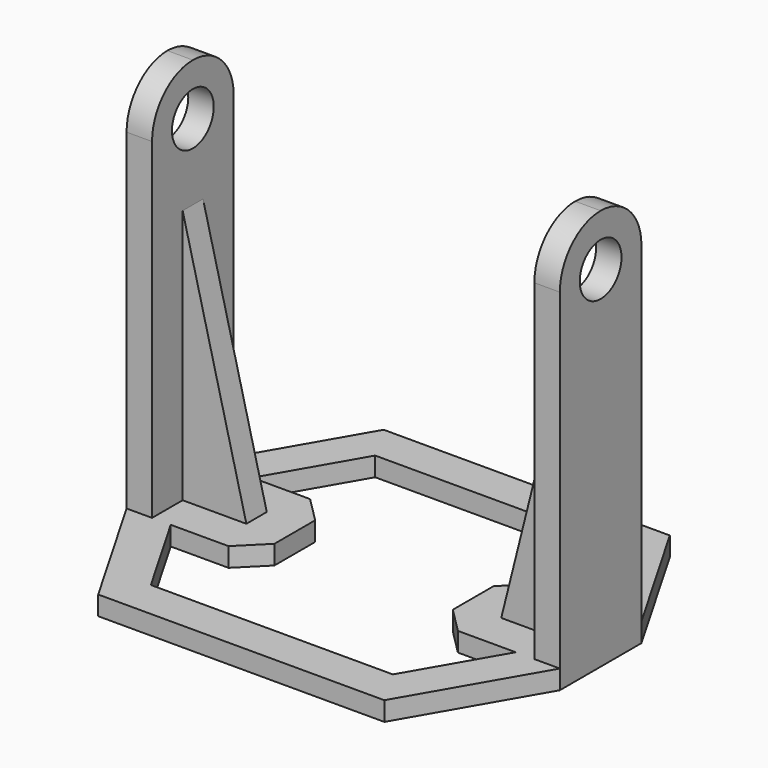
from build123d import *

# Parameters (mm, degrees)
F1_DEPTH = 4
F2_R     = 2.05
F3_DEPTH = 34.001
F5_DEPTH = 1
F7_DEPTH = 1.5
F9_DEPTH = 1.501
F10_SIZE = 2
F11_R    = 3.99999


# Not quite as in the source:
# - a fillet or chamfer is up to 0.001 mm smaller than in the source, because OpenCascade refuses the exact size


with BuildPart() as f1:
    # F0 (on Front) → F1 (new body, symmetric)
    with BuildSketch(Plane.XZ):
        Polygon((15, 0), (0, 0), (-15, 0), (-15, 30), (-17, 30), (-17, -1.5), (0, -1.5), (17, -1.5), (17, 30), (15, 30), align=None)
    extrude(amount=F1_DEPTH, both=True)

    # F2 (on face) → F3 (cut, through all)
    with BuildSketch(Plane.YZ.offset(17)):
        with Locations((0, 25.95)):
            Circle(F2_R)
    extrude(amount=-F3_DEPTH, mode=Mode.SUBTRACT)

    # F4 (on Front) → F5 (join, symmetric)
    with BuildSketch(Plane.XZ):
        Polygon((-10, 0), (-15, 20), (-15, 0), align=None)
        Polygon((15, 20), (10, 0), (15, 0), align=None)
    extrude(amount=F5_DEPTH, both=True)

    # F6 (on face) → F7 (join, through all)
    with BuildSketch(Plane.XY):
        Polygon((15, -4), (-15, -4), (-17, -4), (-11.2264973081, -14), (0, -14), (11.2264973081, -14), (17, -4), align=None)
        Polygon((-11.2264973081, 14), (-17, 4), (-15, 4), (15, 4), (17, 4), (11.2264973081, 14), (0, 14), align=None)
    extrude(amount=-F7_DEPTH)

    # F8 (on face) → F9 (cut, through all)
    with BuildSketch(Plane.XY):
        Polygon((-7, -4), (-13.5358983849, -4), (-9.4944465005, -11), (9.4944465005, -11), (13.5358983849, -4), (7, -4), (7, 4), (13.5358983849, 4), (9.4944465005, 11), (-9.4944465005, 11), (-13.5358983849, 4), (-7, 4), align=None)
    extrude(amount=-F9_DEPTH, mode=Mode.SUBTRACT)

    # F10
    f10_edges = [f1.edges().sort_by_distance(p)[0] for p in [
        (-7, -4, -0.75),
        (-7, 4, -0.75),
        (7, -4, -0.75),
        (7, 4, -0.75),
    ]]
    chamfer(f10_edges, length=F10_SIZE)

    # F11 (radius 4 in the source; OpenCascade refuses exactly that, so slightly less here)
    f11_edges = [f1.edges().sort_by_distance(p)[0] for p in [
        (-16, -4, 30),
        (16, -4, 30),
        (16, 4, 30),
        (-16, 4, 30),
    ]]
    fillet(f11_edges, radius=F11_R)


solid = f1.part
